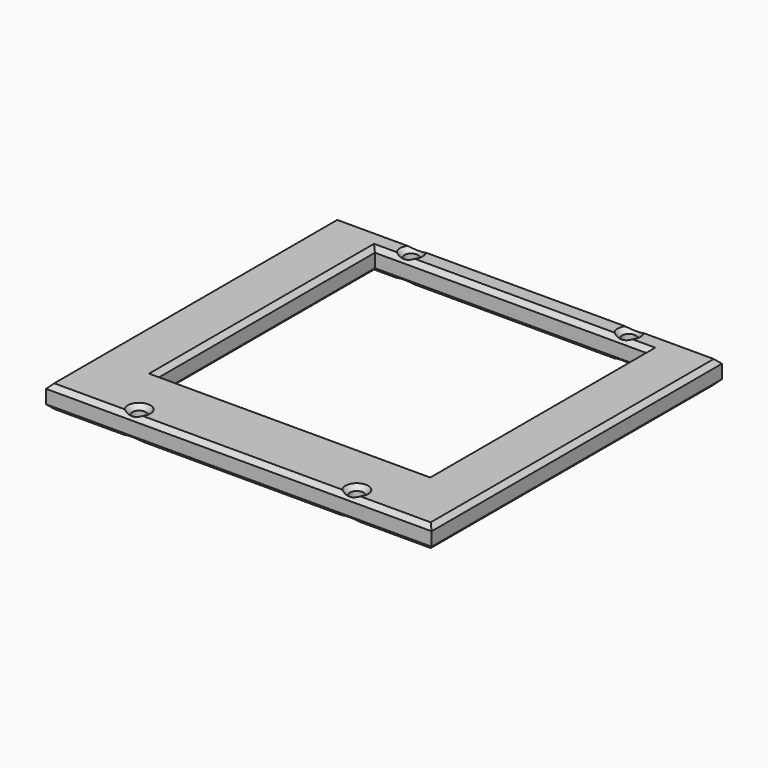
from build123d import *

# Parameters (mm, degrees)
F0_W          = 85
F0_H          = 80
F0_R          = 1.5
F0_W_2        = 60
F0_H_2        = 60
F1_DEPTH      = 5
F2_T1_DEPTH   = 90.1433659759
F2_T3_DEPTH   = 85.1433659759
F2_T5_DEPTH   = 60
F2_T7_DEPTH   = 60
F2_T29_DEPTH  = 62.571682988
F2_T33_DEPTH  = 62.571682988
F2_T40_DEPTH  = 62.571682988
F2_T44_DEPTH  = 62.571682988
F2_T51_DEPTH  = 62.571682988
F2_T55_DEPTH  = 62.571682988
F2_T62_DEPTH  = 62.571682988
F2_T66_DEPTH  = 62.571682988
F2_T73_DEPTH  = 62.571682988
F2_T77_DEPTH  = 62.571682988
F2_T84_DEPTH  = 62.571682988
F2_T88_DEPTH  = 62.571682988
F2_T95_DEPTH  = 62.571682988
F2_T99_DEPTH  = 62.571682988
F2_T106_DEPTH = 62.571682988
F2_T110_DEPTH = 62.571682988


# Not quite as in the source:
# - a fillet or chamfer that OpenCascade refuses, or shapes differently, is made with other operations: its cross-section is extruded or revolved along the edge and cut away or added


with BuildPart() as f1:
    # F0 (on Top) → F1 (new body)
    with BuildSketch(Plane.XY):
        Rectangle(F0_W, F0_H)
        with Locations((-24, -37.5)):
            Circle(F0_R, mode=Mode.SUBTRACT)
        with Locations((24, -37.5)):
            Circle(F0_R, mode=Mode.SUBTRACT)
        with Locations((-24, 37.5)):
            Circle(F0_R, mode=Mode.SUBTRACT)
        with Locations((0, 5)):
            Rectangle(F0_W_2, F0_H_2, mode=Mode.SUBTRACT)
        with Locations((24, 37.5)):
            Circle(F0_R, mode=Mode.SUBTRACT)
    extrude(amount=F1_DEPTH)

    # F2: chamfer of 1 on 24 edges, made by hand

    # F2_s2 → F2_t1 (cut)
    with BuildSketch(Plane.YZ.offset(-45.071682988)):
        Polygon((40, 4), (39, 5), (40, 5), align=None)
        Polygon((-40, 4), (-39, 5), (-40, 5), align=None)
        Polygon((40, 1), (39, 0), (40, 0), align=None)
        Polygon((-40, 1), (-39, 0), (-40, 0), align=None)
    extrude(amount=F2_T1_DEPTH, mode=Mode.SUBTRACT)

    # F2_s4 → F2_t3 (cut)
    with BuildSketch(Plane.XZ.offset(-42.571682988)):
        Polygon((-42.5, 4), (-41.5, 5), (-42.5, 5), align=None)
        Polygon((42.5, 4), (41.5, 5), (42.5, 5), align=None)
        Polygon((-42.5, 1), (-41.5, 0), (-42.5, 0), align=None)
        Polygon((42.5, 1), (41.5, 0), (42.5, 0), align=None)
    extrude(amount=F2_T3_DEPTH, mode=Mode.SUBTRACT)

    # F2_s6 → F2_t5 (cut)
    with BuildSketch(Plane.XZ.offset(-35)):
        Polygon((-30, 4), (-31, 5), (-30, 5), align=None)
        Polygon((30, 4), (31, 5), (30, 5), align=None)
        Polygon((-30, 1), (-31, 0), (-30, 0), align=None)
        Polygon((30, 1), (31, 0), (30, 0), align=None)
    extrude(amount=F2_T5_DEPTH, mode=Mode.SUBTRACT)

    # F2_s8 → F2_t7 (cut)
    with BuildSketch(Plane.YZ.offset(-30)):
        Polygon((35, 4), (36, 5), (35, 5), align=None)
        Polygon((-25, 4), (-26, 5), (-25, 5), align=None)
        Polygon((35, 1), (36, 0), (35, 0), align=None)
        Polygon((-25, 1), (-26, 0), (-25, 0), align=None)
    extrude(amount=F2_T7_DEPTH, mode=Mode.SUBTRACT)

    # F2_s9 → F2_t10 (revolve, cut)
    with BuildSketch(Plane.XZ.offset(37.5)):
        Polygon((-22.5, 4), (-21.5, 5), (-22.5, 5), align=None)
    revolve(axis=Axis((-24, -37.5, 5), (0, 0, 1)), mode=Mode.SUBTRACT)

    # F2_s11 → F2_t12 (revolve, cut)
    with BuildSketch(Plane.XZ.offset(37.5)):
        Polygon((25.5, 4), (26.5, 5), (25.5, 5), align=None)
    revolve(axis=Axis((24, -37.5, 5), (0, 0, 1)), mode=Mode.SUBTRACT)

    # F2_s13 → F2_t14 (revolve, cut)
    with BuildSketch(Plane.XZ.offset(-37.5)):
        Polygon((-22.5, 4), (-21.5, 5), (-22.5, 5), align=None)
    revolve(axis=Axis((-24, 37.5, 5), (0, 0, 1)), mode=Mode.SUBTRACT)

    # F2_s15 → F2_t16 (revolve, cut)
    with BuildSketch(Plane.XZ.offset(-37.5)):
        Polygon((25.5, 4), (26.5, 5), (25.5, 5), align=None)
    revolve(axis=Axis((24, 37.5, 5), (0, 0, 1)), mode=Mode.SUBTRACT)

    # F2_s17 → F2_t18 (revolve, cut)
    with BuildSketch(Plane.XZ.offset(37.5)):
        Polygon((-22.5, 1), (-21.5, 0), (-22.5, 0), align=None)
    revolve(axis=Axis((-24, -37.5, 0), (0, 0, 1)), mode=Mode.SUBTRACT)

    # F2_s19 → F2_t20 (revolve, cut)
    with BuildSketch(Plane.XZ.offset(37.5)):
        Polygon((25.5, 1), (26.5, 0), (25.5, 0), align=None)
    revolve(axis=Axis((24, -37.5, 0), (0, 0, 1)), mode=Mode.SUBTRACT)

    # F2_s21 → F2_t22 (revolve, cut)
    with BuildSketch(Plane.XZ.offset(-37.5)):
        Polygon((-22.5, 1), (-21.5, 0), (-22.5, 0), align=None)
    revolve(axis=Axis((-24, 37.5, 0), (0, 0, 1)), mode=Mode.SUBTRACT)

    # F2_s23 → F2_t24 (revolve, cut)
    with BuildSketch(Plane.XZ.offset(-37.5)):
        Polygon((25.5, 1), (26.5, 0), (25.5, 0), align=None)
    revolve(axis=Axis((24, 37.5, 0), (0, 0, 1)), mode=Mode.SUBTRACT)


with BuildPart() as f2_tool27:
    # F2_s28 → F2_t29 (new body)
    with BuildSketch(Plane.XZ.offset(27.571682988)):
        Polygon((-30, 4), (-31, 5), (-30, 5), align=None)
    extrude(amount=-F2_T29_DEPTH)

    split(bisect_by=Plane.XZ.offset(25), keep=Keep.TOP)


with BuildPart() as f2_tool31:
    # F2_s32 → F2_t33 (new body)
    with BuildSketch(Plane.YZ.offset(30)):
        Polygon((-25, 4), (-26, 5), (-25, 5), align=None)
    extrude(amount=-F2_T33_DEPTH)

    split(bisect_by=Plane.YZ.offset(-30), keep=Keep.BOTTOM)


with BuildPart() as f2_tool27_1:
    add(f2_tool27.part)

    # F2_t35: intersect F2_tool31
    add(f2_tool31.part, mode=Mode.INTERSECT)


with BuildPart() as f1_1:
    add(f1.part)

    # F2_t25: cut F2_tool27
    add(f2_tool27_1.part, mode=Mode.SUBTRACT)


with BuildPart() as f2_tool38:
    # F2_s39 → F2_t40 (new body)
    with BuildSketch(Plane.XZ.offset(25)):
        Polygon((-30, 4), (-31, 5), (-30, 5), align=None)
    extrude(amount=-F2_T40_DEPTH)

    split(bisect_by=Plane.XZ.offset(-35), keep=Keep.BOTTOM)


with BuildPart() as f2_tool42:
    # F2_s43 → F2_t44 (new body)
    with BuildSketch(Plane.YZ.offset(-32.571682988)):
        Polygon((35, 4), (36, 5), (35, 5), align=None)
    extrude(amount=F2_T44_DEPTH)

    split(bisect_by=Plane.YZ.offset(-30), keep=Keep.BOTTOM)


with BuildPart() as f2_tool38_1:
    add(f2_tool38.part)

    # F2_t46: intersect F2_tool42
    add(f2_tool42.part, mode=Mode.INTERSECT)


with BuildPart() as f1_2:
    add(f1_1.part)

    # F2_t36: cut F2_tool38
    add(f2_tool38_1.part, mode=Mode.SUBTRACT)


with BuildPart() as f2_tool49:
    # F2_s50 → F2_t51 (new body)
    with BuildSketch(Plane.YZ.offset(-30)):
        Polygon((35, 4), (36, 5), (35, 5), align=None)
    extrude(amount=F2_T51_DEPTH)

    split(bisect_by=Plane.YZ.offset(30), keep=Keep.TOP)


with BuildPart() as f2_tool53:
    # F2_s54 → F2_t55 (new body)
    with BuildSketch(Plane.XZ.offset(-37.571682988)):
        Polygon((30, 4), (31, 5), (30, 5), align=None)
    extrude(amount=F2_T55_DEPTH)

    split(bisect_by=Plane.XZ.offset(-35), keep=Keep.BOTTOM)


with BuildPart() as f2_tool49_1:
    add(f2_tool49.part)

    # F2_t57: intersect F2_tool53
    add(f2_tool53.part, mode=Mode.INTERSECT)


with BuildPart() as f1_3:
    add(f1_2.part)

    # F2_t47: cut F2_tool49
    add(f2_tool49_1.part, mode=Mode.SUBTRACT)


with BuildPart() as f2_tool60:
    # F2_s61 → F2_t62 (new body)
    with BuildSketch(Plane.XZ.offset(-35)):
        Polygon((30, 4), (31, 5), (30, 5), align=None)
    extrude(amount=F2_T62_DEPTH)

    split(bisect_by=Plane.XZ.offset(25), keep=Keep.TOP)


with BuildPart() as f2_tool64:
    # F2_s65 → F2_t66 (new body)
    with BuildSketch(Plane.YZ.offset(32.571682988)):
        Polygon((-25, 4), (-26, 5), (-25, 5), align=None)
    extrude(amount=-F2_T66_DEPTH)

    split(bisect_by=Plane.YZ.offset(30), keep=Keep.TOP)


with BuildPart() as f2_tool60_1:
    add(f2_tool60.part)

    # F2_t68: intersect F2_tool64
    add(f2_tool64.part, mode=Mode.INTERSECT)


with BuildPart() as f1_4:
    add(f1_3.part)

    # F2_t58: cut F2_tool60
    add(f2_tool60_1.part, mode=Mode.SUBTRACT)


with BuildPart() as f2_tool71:
    # F2_s72 → F2_t73 (new body)
    with BuildSketch(Plane.XZ.offset(27.571682988)):
        Polygon((-30, 1), (-31, 0), (-30, 0), align=None)
    extrude(amount=-F2_T73_DEPTH)

    split(bisect_by=Plane.XZ.offset(25), keep=Keep.TOP)


with BuildPart() as f2_tool75:
    # F2_s76 → F2_t77 (new body)
    with BuildSketch(Plane.YZ.offset(30)):
        Polygon((-25, 1), (-26, 0), (-25, 0), align=None)
    extrude(amount=-F2_T77_DEPTH)

    split(bisect_by=Plane.YZ.offset(-30), keep=Keep.BOTTOM)


with BuildPart() as f2_tool71_1:
    add(f2_tool71.part)

    # F2_t79: intersect F2_tool75
    add(f2_tool75.part, mode=Mode.INTERSECT)


with BuildPart() as f1_5:
    add(f1_4.part)

    # F2_t69: cut F2_tool71
    add(f2_tool71_1.part, mode=Mode.SUBTRACT)


with BuildPart() as f2_tool82:
    # F2_s83 → F2_t84 (new body)
    with BuildSketch(Plane.XZ.offset(25)):
        Polygon((-30, 1), (-31, 0), (-30, 0), align=None)
    extrude(amount=-F2_T84_DEPTH)

    split(bisect_by=Plane.XZ.offset(-35), keep=Keep.BOTTOM)


with BuildPart() as f2_tool86:
    # F2_s87 → F2_t88 (new body)
    with BuildSketch(Plane.YZ.offset(-32.571682988)):
        Polygon((35, 1), (36, 0), (35, 0), align=None)
    extrude(amount=F2_T88_DEPTH)

    split(bisect_by=Plane.YZ.offset(-30), keep=Keep.BOTTOM)


with BuildPart() as f2_tool82_1:
    add(f2_tool82.part)

    # F2_t90: intersect F2_tool86
    add(f2_tool86.part, mode=Mode.INTERSECT)


with BuildPart() as f1_6:
    add(f1_5.part)

    # F2_t80: cut F2_tool82
    add(f2_tool82_1.part, mode=Mode.SUBTRACT)


with BuildPart() as f2_tool93:
    # F2_s94 → F2_t95 (new body)
    with BuildSketch(Plane.YZ.offset(-30)):
        Polygon((35, 1), (36, 0), (35, 0), align=None)
    extrude(amount=F2_T95_DEPTH)

    split(bisect_by=Plane.YZ.offset(30), keep=Keep.TOP)


with BuildPart() as f2_tool97:
    # F2_s98 → F2_t99 (new body)
    with BuildSketch(Plane.XZ.offset(-37.571682988)):
        Polygon((30, 1), (31, 0), (30, 0), align=None)
    extrude(amount=F2_T99_DEPTH)

    split(bisect_by=Plane.XZ.offset(-35), keep=Keep.BOTTOM)


with BuildPart() as f2_tool93_1:
    add(f2_tool93.part)

    # F2_t101: intersect F2_tool97
    add(f2_tool97.part, mode=Mode.INTERSECT)


with BuildPart() as f1_7:
    add(f1_6.part)

    # F2_t91: cut F2_tool93
    add(f2_tool93_1.part, mode=Mode.SUBTRACT)


with BuildPart() as f2_tool104:
    # F2_s105 → F2_t106 (new body)
    with BuildSketch(Plane.XZ.offset(-35)):
        Polygon((30, 1), (31, 0), (30, 0), align=None)
    extrude(amount=F2_T106_DEPTH)

    split(bisect_by=Plane.XZ.offset(25), keep=Keep.TOP)


with BuildPart() as f2_tool108:
    # F2_s109 → F2_t110 (new body)
    with BuildSketch(Plane.YZ.offset(32.571682988)):
        Polygon((-25, 1), (-26, 0), (-25, 0), align=None)
    extrude(amount=-F2_T110_DEPTH)

    split(bisect_by=Plane.YZ.offset(30), keep=Keep.TOP)


with BuildPart() as f2_tool104_1:
    add(f2_tool104.part)

    # F2_t112: intersect F2_tool108
    add(f2_tool108.part, mode=Mode.INTERSECT)


with BuildPart() as f1_8:
    add(f1_7.part)

    # F2_t102: cut F2_tool104
    add(f2_tool104_1.part, mode=Mode.SUBTRACT)


solid = f1_8.part
